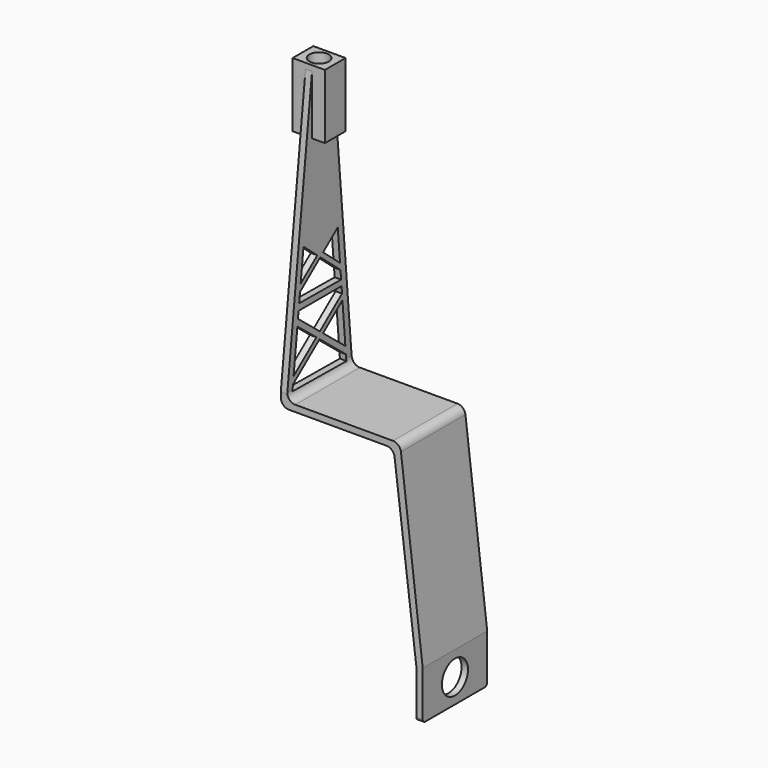
from build123d import *

# Parameters (mm, degrees)
F1_DEPTH     = 50
F3_D         = 20.2
F5_DEPTH     = 25
F6_T1_DEPTH  = 50
F6_T6_DEPTH  = 50
F6_T13_DEPTH = 50
F6_T19_DEPTH = 50
F6_T26_DEPTH = 50
F6_T33_DEPTH = 50
F6_T36_DEPTH = 72.2096061325
F6_T38_DEPTH = 75
F7_T1_DEPTH  = 4.6205948456
F7_T3_DEPTH  = 14
F8_W         = 20
F8_H         = 16
F8_W_2       = 4
F8_H_2       = 15.2079220091
F9_DEPTH     = 40
F10_D        = 12
F10_DEPTH    = 37
F10_TIP      = 3.6051637142


# Not quite as in the source:
# - a fillet or chamfer that OpenCascade refuses, or shapes differently, is made with other operations: its cross-section is extruded or revolved along the edge and cut away or added
# - a feature names something its author has since deleted; it is built from what else it names


with BuildPart() as f1:
    # F0 (on Front) → F1 (new body)
    with BuildSketch(Plane.XZ):
        Polygon((0, 30), (0, 0), (4, 0), (4, 30), (-10.0149744916, 148.1428074388), (-14.0149744916, 148.1428074388), (-80.0149744916, 148.1428074388), (-80.0149744916, 324.1428074388), (-84.0149744916, 324.1428074388), (-84.0149744916, 144.1428074388), (-14.0149744916, 144.1428074388), align=None)
    extrude(amount=F1_DEPTH)

    # F3 (through all)
    with Locations(Plane.YZ.offset(4)):
        with Locations((-25, 15)):
            Hole(F3_D / 2)

    # F4 (on face) → F5 (cut)
    with BuildSketch(Plane.YZ.offset(-80.0149744916)):
        Polygon((-50, 324.1428074388), (-50, 236.1428074388), (-50, 199.9447409799), (-50, 195.9447409799), (-50, 194.2019151126), (-50, 156.2548764067), (-50, 152.2548764067), (-39.9857666554, 240.1486744376), (-30.4158440182, 324.1428074388), align=None)
        Polygon((0, 324.1428074388), (-15.2079220091, 324.1428074388), (-7.806897337, 240.2772722232), (0, 151.8125457081), (0, 244.1428074388), align=None)
        Polygon((-45.5760135212, 155.7661052017), (-45.9782811199, 152.2160466314), (-4.1864533227, 151.8125457081), (-4.5209163536, 155.6025507861), (-24.936375975, 172.1473690272), align=None)
        Polygon((-9.0844288508, 207.3145008204), (-10.8621816933, 227.4593051175), (-22.1599204596, 218.427607474), align=None)
        Polygon((-42.1400031958, 186.0892978758), (-45.0776405527, 160.1643048917), (-27.431660318, 174.1695633191), align=None)
        Polygon((-39.5929888388, 208.4884916623), (-26.7007793174, 218.6382363502), (-37.4004572752, 227.7320942228), align=None)
        Polygon((-22.2456820263, 174.2829185178), (-4.9311455022, 160.2511080648), (-7.2217303873, 186.2071257598), align=None)
        Polygon((-8.7363235607, 203.3699069618), (-24.3721529686, 216.6590929463), (-40.0940653957, 204.0905991656), (-40.7694266569, 198.1630294508), (-8.2490940623, 197.8488116452), align=None)
        Polygon((-41.6920664445, 190.0423920546), (-24.7411634004, 176.305272485), (-7.5520306119, 189.9499595352), (-7.9272601749, 194.2019151126), (-41.2207386286, 194.2019151126), align=None)
    extrude(amount=-F5_DEPTH, mode=Mode.SUBTRACT)

    # F6: fillet of radius 5 on 4 edges, made by hand

    # F6_s2 → F6_t1 (join)
    with BuildSketch(Plane.XZ):
        with BuildLine():
            ThreePointArc((-18.4386008144, 144.1428074388), (-15.1255005733, 142.8875860427), (-13.4758700562, 139.7521541558))
            Line((-13.4758700562, 139.7521541558), (-14.0149744916, 144.1428074388))
            Line((-14.0149744916, 144.1428074388), (-18.4386008144, 144.1428074388))
        make_face()
    extrude(amount=F6_T1_DEPTH)


with BuildPart() as f6_tool4:
    # F6_s5 → F6_t6 (new body)
    with BuildSketch(Plane.XZ):
        with BuildLine():
            ThreePointArc((-80.0149744916, 153.1428074388), (-78.5505083975, 149.6072735328), (-75.0149744916, 148.1428074388))
            Line((-75.0149744916, 148.1428074388), (-80.0149744916, 148.1428074388))
            Line((-80.0149744916, 148.1428074388), (-80.0149744916, 153.1428074388))
        make_face()
    extrude(amount=F6_T6_DEPTH)

    split(bisect_by=Plane(origin=(0, 13.2937308283, 1.1731544977), x_dir=(1, 0, 0), z_dir=(0, -0.9961286805, -0.0879070636)), keep=Keep.TOP)

    split(bisect_by=Plane(origin=(0, 1.465226283, 151.7579786298), x_dir=(1, 0, 0), z_dir=(0, 0.0096545698, 0.9999533936)), keep=Keep.TOP)

    split(bisect_by=Plane(origin=(0, 9.1396289593, 0.8065603975), x_dir=(1, 0, 0), z_dir=(0, 0.9961286805, 0.0879070636)), keep=Keep.TOP)


with BuildPart() as f1_1:
    add(f1.part)

    # F6_t3: union F6_tool4
    add(f6_tool4.part)


with BuildPart() as f6_tool11:
    # F6_s12 → F6_t13 (new body)
    with BuildSketch(Plane.XZ):
        with BuildLine():
            ThreePointArc((-80.0149744916, 153.1428074388), (-78.5505083975, 149.6072735328), (-75.0149744916, 148.1428074388))
            Line((-75.0149744916, 148.1428074388), (-80.0149744916, 148.1428074388))
            Line((-80.0149744916, 148.1428074388), (-80.0149744916, 153.1428074388))
        make_face()
    extrude(amount=F6_T13_DEPTH)

    split(bisect_by=Plane(origin=(0, 1.465226283, 151.7579786298), x_dir=(1, 0, 0), z_dir=(0, -0.0096545698, -0.9999533936)), keep=Keep.TOP)

    split(bisect_by=Plane(origin=(0, 9.1396289593, 0.8065603975), x_dir=(1, 0, 0), z_dir=(0, 0.9961286805, 0.0879070636)), keep=Keep.TOP)


with BuildPart() as f1_2:
    add(f1_1.part)

    # F6_t10: union F6_tool11
    add(f6_tool11.part)


with BuildPart() as f6_tool17:
    # F6_s18 → F6_t19 (new body)
    with BuildSketch(Plane.XZ):
        with BuildLine():
            ThreePointArc((-80.0149744916, 153.1428074388), (-78.5505083975, 149.6072735328), (-75.0149744916, 148.1428074388))
            Line((-75.0149744916, 148.1428074388), (-80.0149744916, 148.1428074388))
            Line((-80.0149744916, 148.1428074388), (-80.0149744916, 153.1428074388))
        make_face()
    extrude(amount=F6_T19_DEPTH)

    split(bisect_by=Plane(origin=(0, -62.4248064238, 7.0735387838), x_dir=(1, 0, 0), z_dir=(0, 0.9936412568, -0.1125924191)), keep=Keep.TOP)

    split(bisect_by=Plane(origin=(0, 1.465226283, 151.7579786298), x_dir=(1, 0, 0), z_dir=(0, -0.0096545698, -0.9999533936)), keep=Keep.TOP)

    split(bisect_by=Plane(origin=(0, 9.1396289593, 0.8065603975), x_dir=(1, 0, 0), z_dir=(0, -0.9961286805, -0.0879070636)), keep=Keep.TOP)


with BuildPart() as f1_3:
    add(f1_2.part)

    # F6_t16: union F6_tool17
    add(f6_tool17.part)


with BuildPart() as f6_tool24:
    # F6_s25 → F6_t26 (new body)
    with BuildSketch(Plane.XZ):
        with BuildLine():
            ThreePointArc((-80.0149744916, 153.1428074388), (-78.5505083975, 149.6072735328), (-75.0149744916, 148.1428074388))
            Line((-75.0149744916, 148.1428074388), (-80.0149744916, 148.1428074388))
            Line((-80.0149744916, 148.1428074388), (-80.0149744916, 153.1428074388))
        make_face()
    extrude(amount=F6_T26_DEPTH)

    split(bisect_by=Plane(origin=(0, -66.484199108, 7.5749176678), x_dir=(1, 0, 0), z_dir=(0, 0.9935718557, -0.1132032138)), keep=Keep.TOP)

    split(bisect_by=Plane(origin=(0, -62.4248064238, 7.0735387838), x_dir=(1, 0, 0), z_dir=(0, -0.9936412568, 0.1125924191)), keep=Keep.TOP)

    split(bisect_by=Plane(origin=(0, 1.465226283, 151.7579786298), x_dir=(1, 0, 0), z_dir=(0, 0.0096545698, 0.9999533936)), keep=Keep.TOP)


with BuildPart() as f1_4:
    add(f1_3.part)

    # F6_t23: union F6_tool24
    add(f6_tool24.part)


with BuildPart() as f6_tool31:
    # F6_s32 → F6_t33 (new body)
    with BuildSketch(Plane.XZ):
        with BuildLine():
            ThreePointArc((-80.0149744916, 153.1428074388), (-78.5505083975, 149.6072735328), (-75.0149744916, 148.1428074388))
            Line((-75.0149744916, 148.1428074388), (-80.0149744916, 148.1428074388))
            Line((-80.0149744916, 148.1428074388), (-80.0149744916, 153.1428074388))
        make_face()
    extrude(amount=F6_T33_DEPTH)

    split(bisect_by=Plane(origin=(0, -62.4248064238, 7.0735387838), x_dir=(1, 0, 0), z_dir=(0, -0.9936412568, 0.1125924191)), keep=Keep.TOP)

    split(bisect_by=Plane(origin=(0, 1.465226283, 151.7579786298), x_dir=(1, 0, 0), z_dir=(0, -0.0096545698, -0.9999533936)), keep=Keep.TOP)


with BuildPart() as f1_5:
    add(f1_4.part)

    # F6_t30: union F6_tool31
    add(f6_tool31.part)

    # F6_s37 → F6_t36 (cut)
    with BuildSketch(Plane.XZ.offset(-11.1048030662)):
        with BuildLine():
            ThreePointArc((-14.4568957181, 148.1428074388), (-11.1361304097, 146.8807905536), (-9.4917098577, 143.7318145454))
            Line((-9.4917098577, 143.7318145454), (-10.0149744916, 148.1428074388))
            Line((-10.0149744916, 148.1428074388), (-14.4568957181, 148.1428074388))
        make_face()
    extrude(amount=F6_T36_DEPTH, mode=Mode.SUBTRACT)

    # F6_s39 → F6_t38 (cut)
    with BuildSketch(Plane.XZ.offset(-12.5)):
        with BuildLine():
            ThreePointArc((-79.0149744916, 144.1428074388), (-82.5505083975, 145.6072735328), (-84.0149744916, 149.1428074388))
            Line((-84.0149744916, 149.1428074388), (-84.0149744916, 144.1428074388))
            Line((-84.0149744916, 144.1428074388), (-79.0149744916, 144.1428074388))
        make_face()
    extrude(amount=F6_T38_DEPTH, mode=Mode.SUBTRACT)

    # F7: fillet of radius 2 on 3 edges, made by hand

    # F7_s2 → F7_t1 (cut)
    with BuildSketch(Plane.YZ.offset(-84.2351683711)):
        with BuildLine():
            ThreePointArc((0, 151.7244681563), (-0.0019365973, 151.8124604227), (-0.007742639, 151.9002822835))
            Line((-0.007742639, 151.9002822835), (0, 151.8125457081))
            Line((0, 151.8125457081), (0, 151.7244681563))
        make_face()
    extrude(amount=F7_T1_DEPTH, mode=Mode.SUBTRACT)

    # F7_s4 → F7_t3 (cut)
    with BuildSketch(Plane.YZ.offset(-5)):
        with BuildLine():
            ThreePointArc((-50, 2), (-49.4142135624, 0.5857864376), (-48, 0))
            Line((-48, 0), (-50, 0))
            Line((-50, 0), (-50, 2))
        make_face()
        with BuildLine():
            ThreePointArc((0, 2), (-0.5857864376, 0.5857864376), (-2, 0))
            Line((-2, 0), (0, 0))
            Line((0, 0), (0, 2))
        make_face()
    extrude(amount=F7_T3_DEPTH, mode=Mode.SUBTRACT)

    # F8 (on face) → F9 (join)
    with BuildSketch(Plane.XY.offset(324.1428074388)):
        with Locations((-82.0149744916, -22.8118830136)):
            Rectangle(F8_W, F8_H)
        with Locations((-82.0149744916, -22.8118830136)):
            Rectangle(F8_W_2, F8_H_2, mode=Mode.SUBTRACT)
    extrude(amount=-F9_DEPTH)

    # F10
    with Locations(Plane.XY.offset(324.1428074388)):
        with Locations((-82.0149744916, -22.8118830136)):
            Hole(F10_D / 2, depth=F10_DEPTH)
            with Locations((0, 0, -(F10_DEPTH + F10_TIP / 2))):  # 118° drill point
                Cone(0, F10_D / 2, F10_TIP, mode=Mode.SUBTRACT)


solid = f1_5.part
